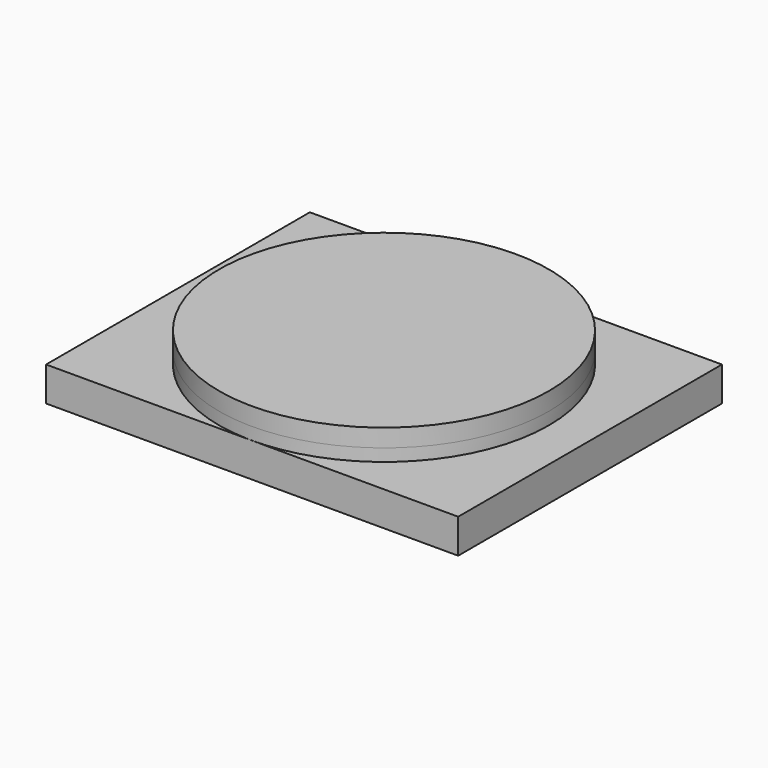
from build123d import *

# Parameters (mm, degrees)
F0_R     = 120
F0_R_2   = 100
F1_DEPTH = 9
F2_DEPTH = 4
F3_DEPTH = 13
F4_DEPTH = 9
F6_DEPTH = 25


with BuildPart() as f1:
    # F0 (on Top) → F1 (new body)
    with BuildSketch(Plane.XY):
        Circle(F0_R)
        Circle(F0_R_2, mode=Mode.SUBTRACT)
        Circle(F0_R_2)
    extrude(amount=-F1_DEPTH)

    # F0 (on Top) → F3 (join)
    with BuildSketch(Plane.XY):
        Circle(F0_R)
        Circle(F0_R_2, mode=Mode.SUBTRACT)
    extrude(amount=F3_DEPTH)



with BuildPart() as f2:
    # F0 (on Top) → F2 (new body)
    with BuildSketch(Plane.XY):
        Circle(F0_R_2)
    extrude(amount=F2_DEPTH)


with BuildPart() as f1_1:
    add(f1.part)
    # F4 (add): a face of the model
    f4_faces = [f2.part.faces().sort_by_distance(p)[0] for p in [
        (0, 0, 4),
    ]]
    extrude(f4_faces, amount=F4_DEPTH)


with BuildPart() as f6:
    # F5 (on face) → F6 (new body)
    with BuildSketch(Plane(origin=(0, 0, -9), x_dir=(1, 0, 0), z_dir=(0, 0, -1))):
        with BuildLine():
            Line((150, -120), (150, 120))
            Line((150, 120), (0, 120))
            ThreePointArc((0, 120), (84.8528137424, 84.8528137424), (120, 0))
            ThreePointArc((120, 0), (84.8528137424, -84.8528137424), (0, -120))
            Line((0, -120), (150, -120))
        make_face()
        with BuildLine():
            ThreePointArc((0, -120), (-120, 0), (0, 120))
            Line((0, 120), (-150, 120))
            Line((-150, 120), (-150, -120))
            Line((-150, -120), (0, -120))
        make_face()
        with BuildLine():
            ThreePointArc((120, 0), (84.8528137424, 84.8528137424), (0, 120))
            ThreePointArc((0, 120), (-120, 0), (0, -120))
            ThreePointArc((0, -120), (84.8528137424, -84.8528137424), (120, 0))
        make_face()
    extrude(amount=F6_DEPTH)


solid = Compound([f2.part, f1_1.part, f6.part])
